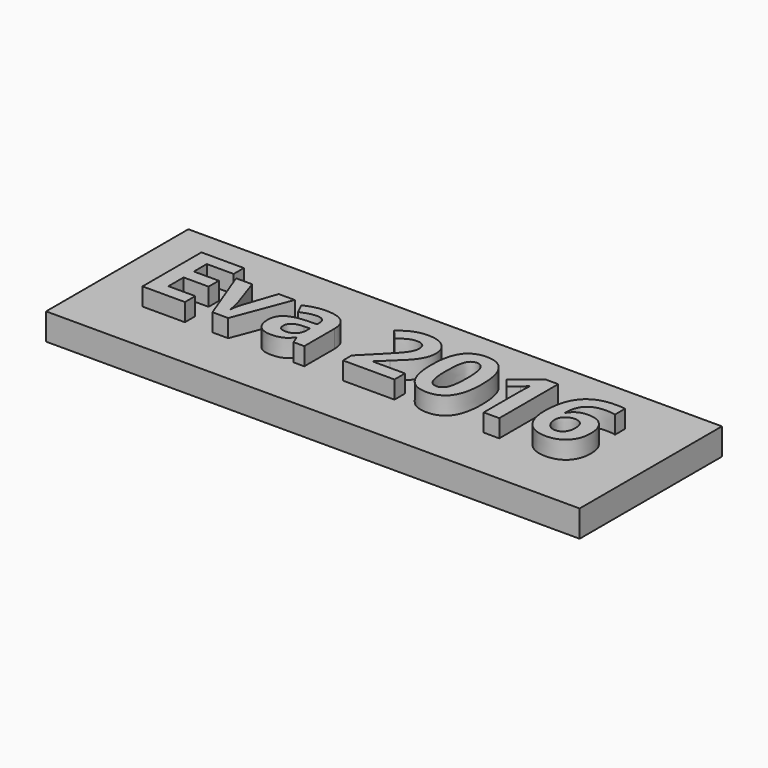
from build123d import *

# Parameters (mm, degrees)
F0_W         = 60
F0_H         = 20
F1_DEPTH     = 3
F2_TEXT_SIZE = 11.603452027
F3_DEPTH     = 2


# Not quite as in the source:
# - Text() gives the source's letters only with a copy of the font that has no kerning and outlines rounded to 1/6400 em; it was checked with that copy


with BuildPart() as f1:
    # F0 (on Top) → F1 (new body)
    with BuildSketch(Plane.XY):
        with Locations((-3.7512257695, -19.1832038106)):
            Rectangle(F0_W, F0_H)
    extrude(amount=F1_DEPTH)

    # F2 (on face) → F3 (join)
    with BuildSketch(Plane.XY.offset(3)):
        with Locations((-28.7512257695, -23.1832038106)):
            Text('Eva 2016', F2_TEXT_SIZE, font='Open Sans', font_style=FontStyle.BOLD, text_align=(TextAlign.LEFT, TextAlign.BOTTOM))
    extrude(amount=F3_DEPTH)


solid = f1.part
